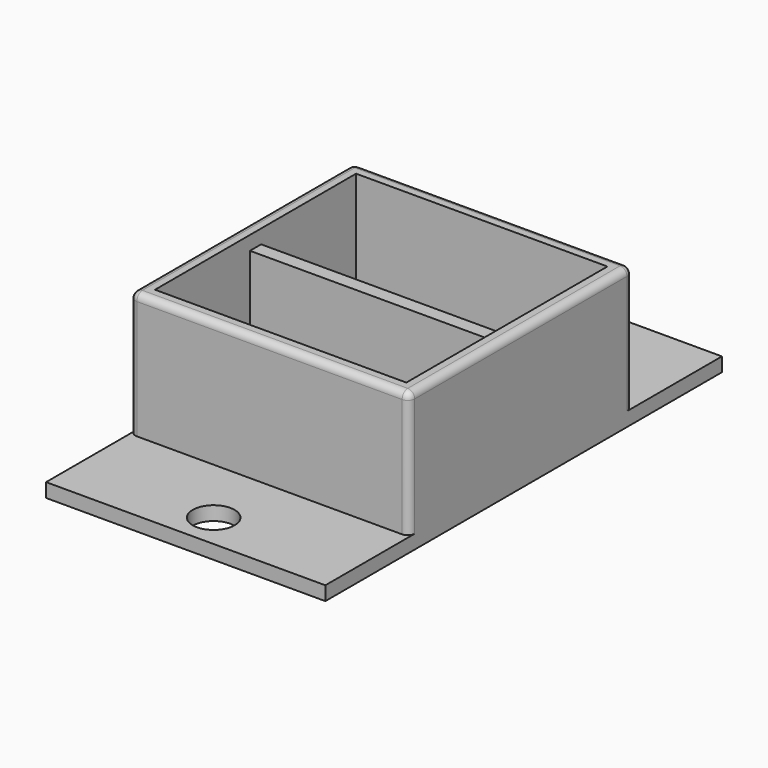
from build123d import *

# Parameters (mm, degrees)
F0_W     = 20
F0_H     = 20
F1_DEPTH = 10
F2_T     = -1
F4_DEPTH = 9
F5_W     = 20
F5_H     = 8
F5_R     = 1.5
F6_DEPTH = 1
F7_W     = 18
F7_H     = 18
F8_DEPTH = 1
F9_R     = 0.5


with BuildPart() as f1:
    # F0 (on Top) → F1 (new body)
    with BuildSketch(Plane.XY):
        Rectangle(F0_W, F0_H)
    extrude(amount=F1_DEPTH)

    # F2
    f2_openings = [f1.faces().sort_by_distance(p)[0] for p in [
        (0, 0, 0),
    ]]
    offset(amount=F2_T, openings=f2_openings)

    # F3 (on Top) → F4 (join)
    with BuildSketch(Plane.XY):
        Polygon((9, -0.5), (9, 0.5), (0.5, 0.5), (-0.5, 0.5), (-9, 0.5), (-9, -0.5), (-0.5, -0.5), (0.5, -0.5), align=None)
    extrude(amount=F4_DEPTH)

    # F5 (on Top) → F6 (join)
    with BuildSketch(Plane.XY):
        with Locations((0, -13.5)):
            Rectangle(F5_W, F5_H)
        with Locations((0, -15)):
            Circle(F5_R, mode=Mode.SUBTRACT)
        with Locations((0, 14)):
            Rectangle(F5_W, F5_H)
        with Locations((0, 15)):
            Circle(F5_R, mode=Mode.SUBTRACT)
    extrude(amount=F6_DEPTH)

    # F7 (on face) → F8 (cut)
    with BuildSketch(Plane.XY.offset(10)):
        Rectangle(F7_W, F7_H)
    extrude(amount=-F8_DEPTH, mode=Mode.SUBTRACT)

    # F9
    f9_edges = [f1.edges().sort_by_distance(p)[0] for p in [
        (-10, -10, 5.5),
        (10, -10, 5.5),
        (0, -10, 10),
        (10, 0, 10),
        (-10, 0, 10),
        (10, 10, 5.5),
        (-10, 10, 5.5),
        (0, 10, 10),
    ]]
    fillet(f9_edges, radius=F9_R)


solid = f1.part
